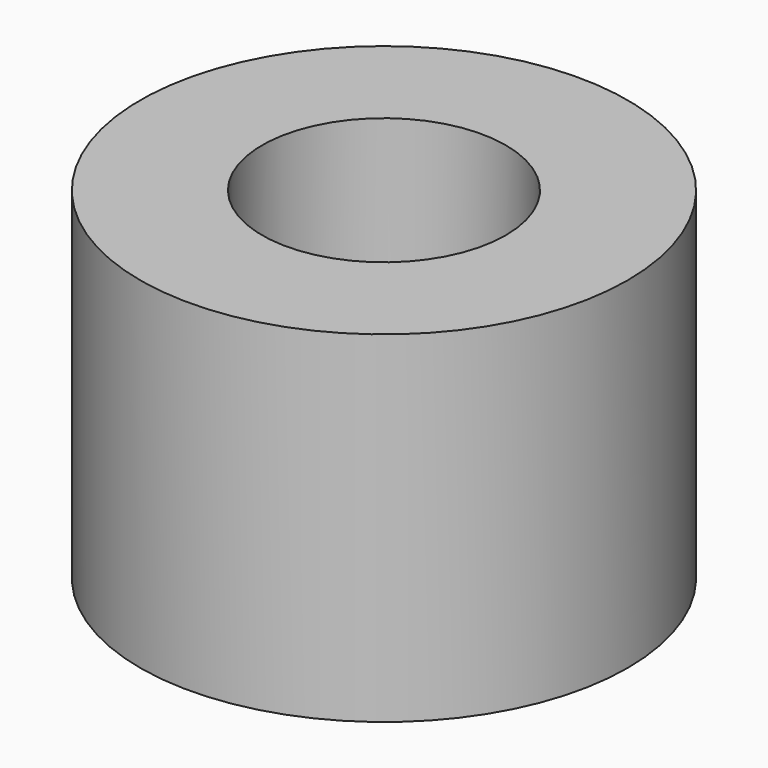
from build123d import *

# Parameters (mm, degrees)
F1_R     = 5
F1_R_2   = 2.5
F2_DEPTH = 7


with BuildPart() as f2:
    # F1 (on Top) → F2 (new body)
    with BuildSketch(Plane.XY):
        Circle(F1_R)
        Circle(F1_R_2, mode=Mode.SUBTRACT)
    extrude(amount=F2_DEPTH)


solid = f2.part
